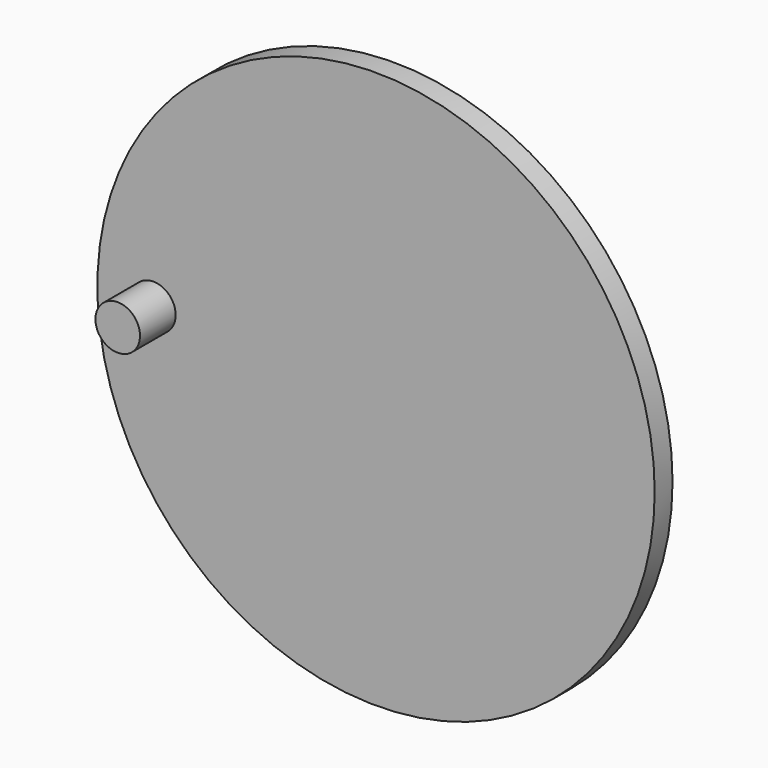
from build123d import *

# Parameters (mm, degrees)
F0_R     = 3175
F1_DEPTH = 127
F2_R     = 254
F3_DEPTH = 508
F4_R     = 254
F5_DEPTH = 762
F7_DEPTH = 381


# Not quite as in the source:
# - a feature names something its author has since deleted; it is built from what else it names


with BuildPart() as f1:
    # F0 (on Front) → F1 (new body, symmetric)
    with BuildSketch(Plane.XZ):
        Circle(F0_R)
    extrude(amount=F1_DEPTH, both=True)

    # F2 (on face) → F3 (join)
    with BuildSketch(Plane.XZ.offset(127)):
        with Locations((-2536.9496234023, 0)):
            Circle(F2_R)
    extrude(amount=F3_DEPTH)

    # F4 (on face) → F5 (join)
    with BuildSketch(Plane(origin=(0, 127, 0), x_dir=(-1, 0, 0), z_dir=(0, 1, 0))):
        Circle(F4_R)
    extrude(amount=F5_DEPTH)

    # F6 (on face) → F7 (cut)
    with BuildSketch(Plane(origin=(0, 889, 0), x_dir=(-1, 0, 0), z_dir=(0, 1, 0))):
        Polygon((173.7058100278, 56.4404390281), (0, 182.6450973749), (-173.7058100278, 56.4404390281), (-107.3560946405, -147.7629877156), (107.3560946405, -147.7629877156), align=None)
    extrude(amount=-F7_DEPTH, mode=Mode.SUBTRACT)


solid = f1.part
